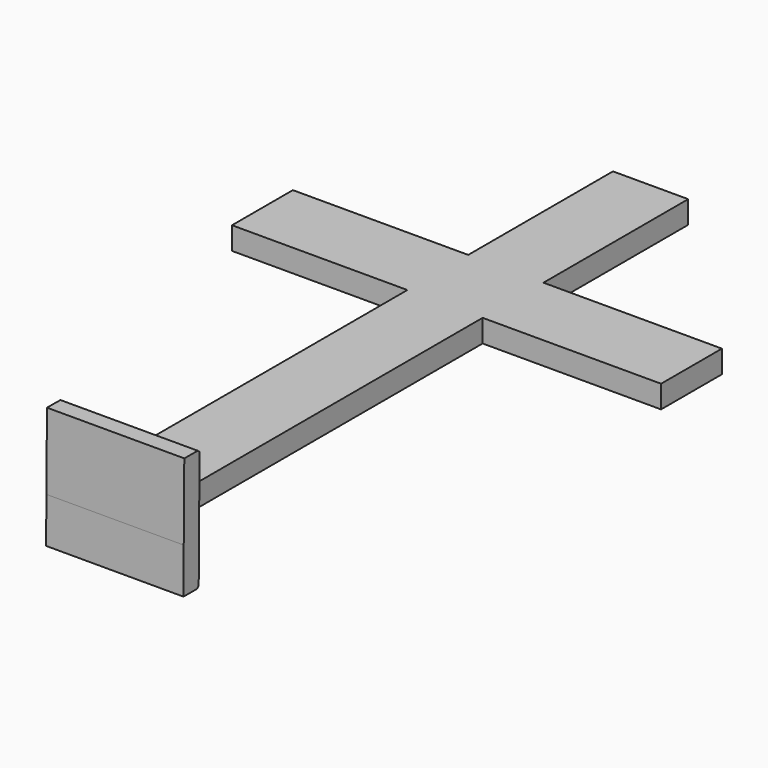
from build123d import *

# Parameters (mm, degrees)
F1_DEPTH    = 2.75
F3_DEPTH    = 16.7
F4_C1_SIZE2 = 2.852938746
F4_C1_SIZE  = 3.4
F4_C2_SIZE2 = 2.852938746
F4_C2_SIZE  = 3.4


with BuildPart() as f1:
    # F0 (on Top) → F1 (new body, symmetric)
    with BuildSketch(Plane.XY):
        Polygon((9.15, 81.3), (0, 81.3), (-9.15, 81.3), (-9.15, 37.3), (-51.8, 37.3), (-51.8, 18.8), (-9.15, 18.8), (-9.15, -81.2), (0, -81.2), (9.15, -81.2), (9.15, 18.8), (52.55, 18.8), (52.55, 37.3), (9.15, 37.3), align=None)
    extrude(amount=F1_DEPTH, both=True)

    # F2 (on Right) → F3 (join, symmetric)
    with BuildSketch(Plane.YZ):
        Polygon((-74.0734412255, -10.8967302314), (-74, -2.75), (-73.8589504462, 12.8964254994), (-77.2330946452, 15.7798974367), (-81.3329280584, 15.8168566562), (-81.4996952681, -2.6823916718), (-81.5988541495, -13.6819447316), (-77.4990207363, -13.718903951), align=None)
    extrude(amount=F3_DEPTH, both=True)

    # F4: chamfer of 3.4 x 2.852938746 on 2 edges, made by hand

    # F4_c1
    f4_c1_edges = [f1.edges().sort_by_distance(p)[0] for p in [
        (-16.7, -73.9661958359, 0.999847634),
    ]]
    f4_c1_side = f1.faces().sort_by_distance((-16.6429412251, -73.9661958359, 0.999847634))[0]
    chamfer(f4_c1_edges, length=F4_C1_SIZE, length2=F4_C1_SIZE2, reference=f4_c1_side)

    # F4_c2
    f4_c2_edges = [f1.edges().sort_by_distance(p)[0] for p in [
        (16.7, -73.9661958359, 0.999847634),
    ]]
    f4_c2_side = f1.faces().sort_by_distance((16.6429412251, -73.9661958359, 0.999847634))[0]
    chamfer(f4_c2_edges, length=F4_C2_SIZE, length2=F4_C2_SIZE2, reference=f4_c2_side)


solid = f1.part
